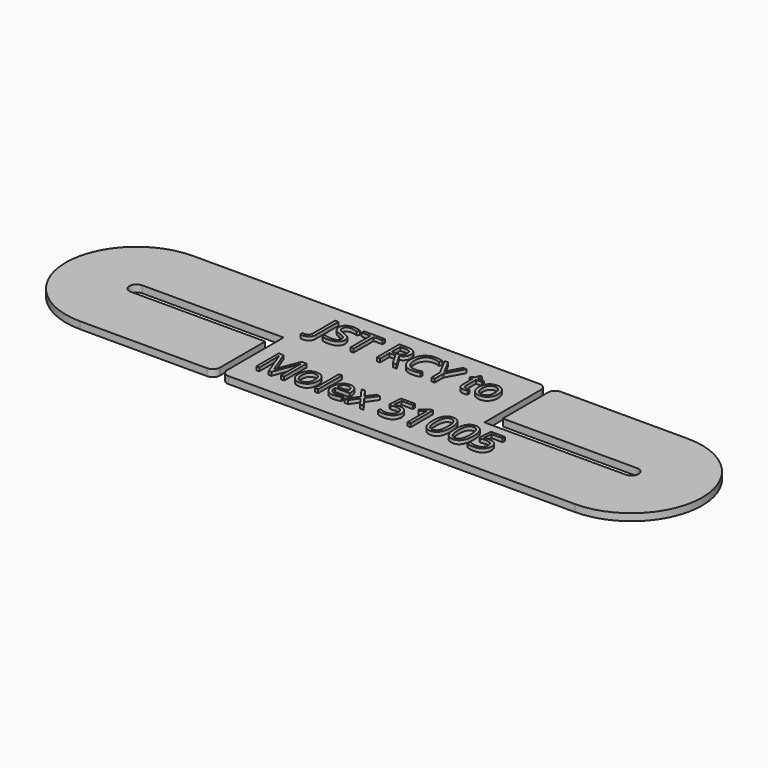
from build123d import *

# Parameters (mm, degrees)
F1_DEPTH     = 1
F2_TEXT_SIZE = 5.5555555556
F3_DEPTH     = 0.5


# Not quite as in the source:
# - Text() gives the source's letters only with a copy of the font that has no kerning and outlines rounded to 1/6400 em; it was checked with that copy


with BuildPart() as f1:
    # F0 (on Top) → F1 (new body)
    with BuildSketch(Plane.XY):
        with BuildLine():
            Line((14, 10), (-15, 10))
            Line((-15, 10), (-15, 1))
            Line((-15, 1), (-15, -9))
            ThreePointArc((-15, -9), (-14.7071067812, -9.7071067812), (-14, -10))
            Line((-14, -10), (15, -10))
            Line((15, -10), (15, -1))
            Line((15, -1), (15, 9))
            ThreePointArc((15, 9), (14.7071067812, 9.7071067812), (14, 10))
        make_face()
        with BuildLine():
            Line((-15, 1), (-15, 10))
            Line((-15, 10), (-35, 10))
            ThreePointArc((-35, 10), (-45, 0), (-35, -10))
            Line((-35, -10), (-17, -10))
            ThreePointArc((-17, -10), (-16.2928932188, -9.7071067812), (-16, -9))
            Line((-16, -9), (-16, -1))
            Line((-16, -1), (-35, -1))
            ThreePointArc((-35, -1), (-36, 0), (-35, 1))
            Line((-35, 1), (-15, 1))
        make_face()
        with BuildLine():
            Line((35, -1), (15, -1))
            Line((15, -1), (15, -10))
            Line((15, -10), (35, -10))
            ThreePointArc((35, -10), (45, 0), (35, 10))
            Line((35, 10), (17, 10))
            ThreePointArc((17, 10), (16.2928932188, 9.7071067812), (16, 9))
            Line((16, 9), (16, 1))
            Line((16, 1), (35, 1))
            ThreePointArc((35, 1), (36, 0), (35, -1))
        make_face()
    extrude(amount=F1_DEPTH)

    # F2 (on face) → F3 (join)
    with BuildSketch(Plane.XY.offset(1)):
        with Locations((-13, 3)):
            Text('JST RCY to', F2_TEXT_SIZE, font='Open Sans', text_align=(TextAlign.LEFT, TextAlign.BOTTOM))
        with Locations((-13, -7)):
            Text('Molex 51005', F2_TEXT_SIZE, font='Open Sans', text_align=(TextAlign.LEFT, TextAlign.BOTTOM))
    extrude(amount=F3_DEPTH)


solid = f1.part
